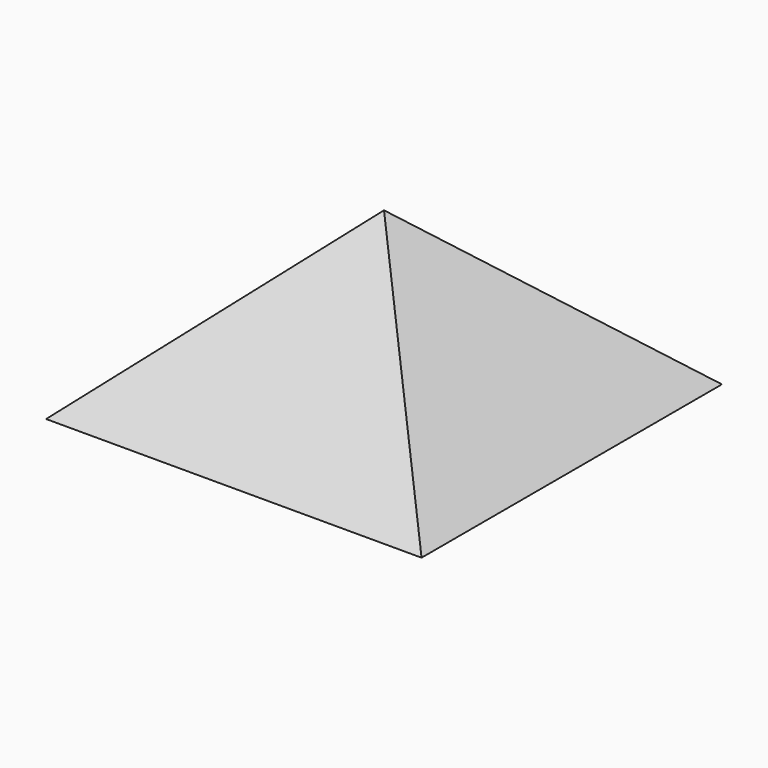
from build123d import *

# Parameters (mm, degrees)
F0_W     = 550
F0_H     = 550
F1_DEPTH = 246.83
F2_SIZE2 = 246.82999
F2_SIZE  = 274.99999
F4_DEPTH = 275


# Not quite as in the source:
# - a fillet or chamfer is up to 0.001 mm smaller than in the source, because OpenCascade refuses the exact size


with BuildPart() as f1:
    # F0 (on Top) → F1 (new body)
    with BuildSketch(Plane.XY):
        Rectangle(F0_W, F0_H)
    extrude(amount=F1_DEPTH)

    # F2 (size 275 and 246.83 in the source; OpenCascade refuses exactly that, so slightly less here)
    f2_edges = [f1.edges().sort_by_distance(p)[0] for p in [
        (0, -275, 246.83),
        (0, 275, 246.83),
    ]]
    f2_side = f1.faces().sort_by_distance((0, 0, 246.83))[0]
    chamfer(f2_edges, length=F2_SIZE, length2=F2_SIZE2, reference=f2_side)

    # F3 (on Front) → F4 (cut, symmetric)
    with BuildSketch(Plane.XZ):
        Polygon((-275, 246.83), (-275, 0), (0, 246.83), align=None)
        Polygon((275, 246.83), (0, 246.83), (275, 0), align=None)
    extrude(amount=F4_DEPTH, both=True, mode=Mode.SUBTRACT)


solid = f1.part
